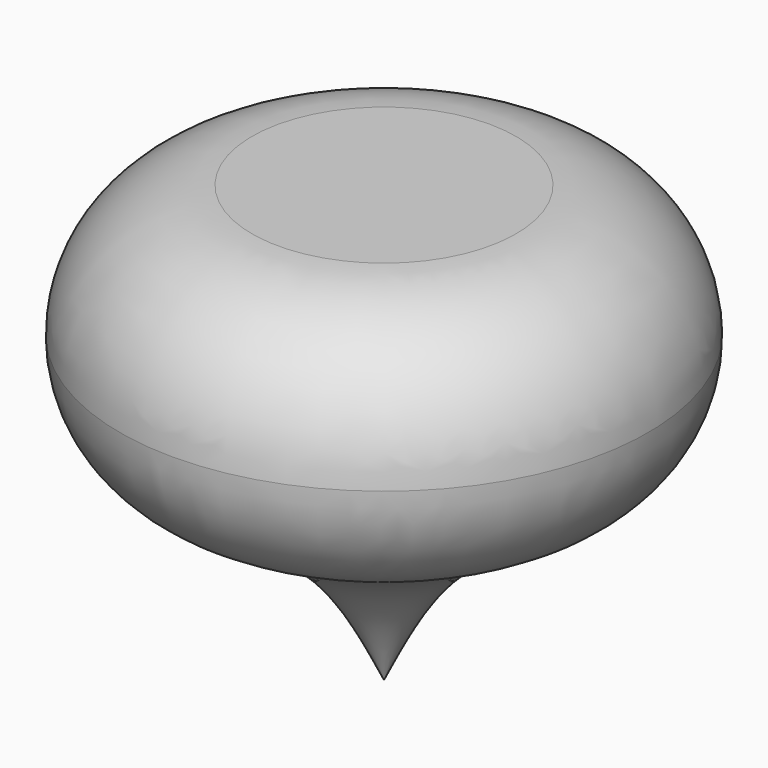
from build123d import *


with BuildPart() as f1:
    # F0 (on Right) → F1 (revolve)
    with BuildSketch(Plane.YZ):
        with BuildLine():
            ThreePointArc((23.4314106154, 33.6637578056), (29.5126985507, 39.4991890718), (31.75, 47.625))
            ThreePointArc((31.75, 47.625), (27.1003201513, 58.8503201513), (15.875, 63.5))
            ThreePointArc((15.875, 63.5), (4.6496797864, 58.8503200891), (0, 47.624999824))
            ThreePointArc((0, 47.624999824), (4.6496799109, 36.3996797864), (15.875, 31.75))
            ThreePointArc((15.875, 31.75), (19.3699927872, 32.1395019319), (22.6934824006, 33.2888944356))
            add(Edge.make_bspline(
                [(22.6934824006, 33.2888944356), (22.9393750786, 33.4138915107), (23.1853973333, 33.5388167735), (23.4314106154, 33.6637578056)],
                knots=[0.9775156082, 0.9775156082, 0.9775156082, 0.9775156082, 1, 1, 1, 1], degree=3))
        make_face()
        with BuildLine():
            ThreePointArc((0, 47.624999824), (4.6496797864, 58.8503200891), (15.875, 63.5))
            Line((15.875, 63.5), (0, 63.5))
            Line((0, 63.5), (0, 47.624999824))
        make_face()
        with BuildLine():
            ThreePointArc((15.875, 31.75), (4.6496799109, 36.3996797864), (0, 47.624999824))
            Line((0, 47.624999824), (0, 11.1125))
            add(Edge.make_bspline(
                [(0, 11.1125), (2.1673627178, 15.6458601549), (6.6288038262, 24.988679858), (17.1930463797, 30.4928029871), (22.6934824006, 33.2888944356)],
                knots=[0, 0, 0, 0, 0.4745565147, 0.9775156082, 0.9775156082, 0.9775156082, 0.9775156082], degree=3))
            ThreePointArc((22.6934824006, 33.2888944356), (19.3699927872, 32.1395019319), (15.875, 31.75))
        make_face()
    revolve(axis=Axis((0, 0, 37.30625), (0, 0, 1)))


solid = f1.part
